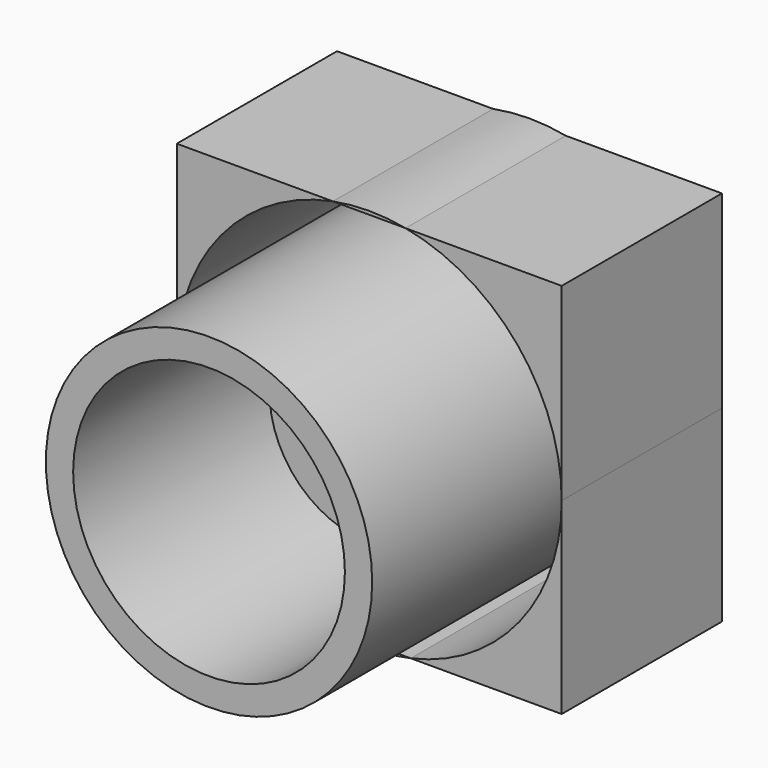
from build123d import *

# Parameters (mm, degrees)
F1_DEPTH = 25.4
F0_R     = 12.6394393626
F0_R_2   = 8.3728331527
F0_R_3   = 5.1773172291
F0_R_4   = 20.6953225865
F0_R_5   = 17.2335435778
F2_DEPTH = 25.4


# Not quite as in the source:
# - ends of sketch curves that miss each other by under 0.0002 mm in the source are joined
# - a feature names something its author has since deleted; it is built from what else it names


with BuildPart() as f1:
    # F0 (on Front) → F1 (new body)
    with BuildSketch(Plane.XZ):
        with BuildLine():
            Line((-12.9094741786, 24.4382098317), (-32.717242837, 24.4382098317))
            Line((-32.717242837, 24.4382098317), (-32.717242837, 0.4653259821))
            ThreePointArc((-32.717242837, 0.4653259821), (-27.1246627125, 16.0140143217), (-12.9094741786, 24.4382098317))
        make_face()
    extrude(amount=F1_DEPTH)


with BuildPart() as f1b:
    # F0 (on Front) → F1, piece 2 (new body)
    with BuildSketch(Plane.XZ):
        with BuildLine():
            ThreePointArc((-13.5706461069, -23.3711004257), (-27.3378712415, -14.8216567814), (-32.7172422573, 0.4653259821))
            Line((-32.7172422573, 0.4653259821), (-32.717242837, -23.3711004257))
            Line((-32.717242837, -23.3711004257), (-13.5706461069, -23.3711004257))
        make_face()
    extrude(amount=F1_DEPTH)


with BuildPart() as f1c:
    # F0 (on Front) → F1, piece 3 (new body)
    with BuildSketch(Plane.XZ):
        with BuildLine():
            ThreePointArc((-3.7034150665, 24.4382098317), (-8.3064446226, 24.8761236168), (-12.9094741786, 24.4382098317))
            Line((-12.9094741786, 24.4382098317), (-3.7034150665, 24.4382098317))
        make_face()
    extrude(amount=F1_DEPTH)


with BuildPart() as f1d:
    # F0 (on Front) → F1, piece 4 (new body)
    with BuildSketch(Plane.XZ):
        with BuildLine():
            Line((16.1043517292, 24.4382098317), (-3.7034150665, 24.4382098317))
            ThreePointArc((-3.7034150665, 24.4382098317), (10.5117734674, 16.0140143217), (16.1043530121, 0.4653259821))
            Line((16.1043530121, 0.4653259821), (16.1043517292, 24.4382098317))
        make_face()
    extrude(amount=F1_DEPTH)


with BuildPart() as f1e:
    # F0 (on Front) → F1, piece 5 (new body)
    with BuildSketch(Plane.XZ):
        with BuildLine():
            ThreePointArc((16.1043530121, 0.4653259821), (10.7249819964, -14.8216567814), (-3.0422431382, -23.3711004257))
            Line((-3.0422431382, -23.3711004257), (16.1043517292, -23.3711004257))
            Line((16.1043517292, -23.3711004257), (16.1043530121, 0.4653259821))
        make_face()
    extrude(amount=F1_DEPTH)


with BuildPart() as f1f:
    # F0 (on Front) → F1, piece 6 (new body)
    with BuildSketch(Plane.XZ):
        with BuildLine():
            Line((-3.0422431382, -23.3711004257), (-13.5706461069, -23.3711004257))
            ThreePointArc((-13.5706461069, -23.3711004257), (-8.3064446226, -23.9454716526), (-3.0422431382, -23.3711004257))
        make_face()
    extrude(amount=F1_DEPTH)


with BuildPart() as f1g:
    # F0 (on Front) → F1, piece 7 (new body)
    with BuildSketch(Plane.XZ):
        with Locations((-8.3064446226, 0.4653259821)):
            Circle(F0_R)
        with Locations((-8.3064446226, 0.4653259821)):
            Circle(F0_R_2, mode=Mode.SUBTRACT)
    extrude(amount=F1_DEPTH)


with BuildPart() as f1h:
    # F0 (on Front) → F1, piece 8 (new body)
    with BuildSketch(Plane.XZ):
        with Locations((-8.3064446226, 0.4653259821)):
            Circle(F0_R_3)
    extrude(amount=F1_DEPTH)


with BuildPart() as f1i:
    # F0 (on Front) → F1, piece 9 (new body)
    with BuildSketch(Plane.XZ):
        with Locations((-8.3064446226, 0.4653259821)):
            Circle(F0_R_4)
        with Locations((-8.3064446226, 0.4653259821)):
            Circle(F0_R_5, mode=Mode.SUBTRACT)
    extrude(amount=F1_DEPTH)

    # F2 (add): a face of the model
    f2_faces = [f1i.faces().sort_by_distance(p)[0] for p in [
        (-28.4164150914, -25.4, 0.4653259821),
    ]]
    extrude(f2_faces, amount=F2_DEPTH)


solid = Compound([f1.part, f1b.part, f1c.part, f1d.part, f1e.part, f1f.part, f1g.part, f1h.part, f1i.part])
